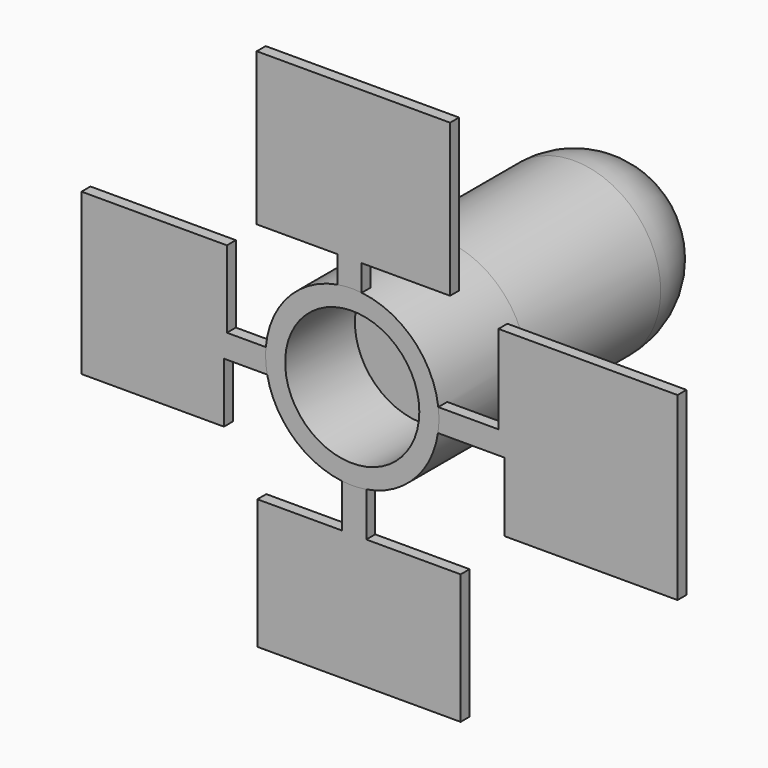
from build123d import *

# Parameters (mm, degrees)
F0_R      = 7.75
F0_R_2    = 5.75
F1_DEPTH  = 7.75
F2_R      = 7.74999
F3_DEPTH  = 15
F4_DEPTH  = 5
F6_R      = 7.75
F6_R_2    = 6
F7_DEPTH  = 9.8
F6_R_3    = 5.75
F8_DEPTH  = 2
F10_DEPTH = 1


# Not quite as in the source:
# - a fillet or chamfer that OpenCascade refuses, or shapes differently, is made with other operations: its cross-section is extruded or revolved along the edge and cut away or added
# - a fillet or chamfer is up to 0.001 mm smaller than in the source, because OpenCascade refuses the exact size


with BuildPart() as f1:
    # F0 (on Front) → F1 (new body)
    with BuildSketch(Plane.XZ):
        Circle(F0_R)
        Circle(F0_R_2, mode=Mode.SUBTRACT)
        Circle(F0_R_2)
    extrude(amount=-F1_DEPTH)

    # F2 (radius 7.75 in the source; OpenCascade refuses exactly that, so slightly less here)
    f2_edges = [f1.edges().sort_by_distance(p)[0] for p in [
        (-7.75, 7.75, 0),
    ]]
    fillet(f2_edges, radius=F2_R)

    # F0 (on Front) → F3 (join)
    with BuildSketch(Plane.XZ):
        Circle(F0_R)
        Circle(F0_R_2, mode=Mode.SUBTRACT)
    extrude(amount=F3_DEPTH)

    # F0 (on Front) → F4 (cut)
    with BuildSketch(Plane.XZ):
        Circle(F0_R_2)
    extrude(amount=-F4_DEPTH, mode=Mode.SUBTRACT)

    # F5: fillet of radius 5.75 on 1 edges, made by hand

    # F5_s1 → F5_t2 (revolve)
    with BuildSketch(Plane.XY):
        with BuildLine():
            ThreePointArc((5.7501, -0.7499), (4.0659639918, 3.3159639918), (0.0001, 5.0001))
            Line((0.0001, 5.0001), (0.0001, 5.1151))
            ThreePointArc((0.0001, 5.1151), (2.87505, 5.115), (5.75, 5.115))
            Line((5.75, 5.115), (5.865, 5))
            ThreePointArc((5.865, 5), (5.865, 2.12505), (5.8651, -0.7499))
            Line((5.8651, -0.7499), (5.7501, -0.7499))
        make_face()
    revolve(axis=Axis((0, 5, 0), (0, -1, 0)))

    # F6 (on face) → F7 (join)
    with BuildSketch(Plane.XZ.offset(15)):
        Circle(F6_R)
        Circle(F6_R_2, mode=Mode.SUBTRACT)
    extrude(amount=F7_DEPTH)

    # F6 (on face) → F8 (join)
    with BuildSketch(Plane.XZ.offset(15)):
        Circle(F6_R_2)
        Circle(F6_R_3, mode=Mode.SUBTRACT)
        Circle(F6_R_3)
    extrude(amount=F8_DEPTH)

    # F9 (on face) → F10 (join)
    with BuildSketch(Plane.XZ.offset(24.8)):
        with BuildLine():
            ThreePointArc((-7.6053065566, -1.4905744465), (-7.7379420075, -0.4321498454), (-7.7239859171, 0.6344616239))
            Line((-7.7239859171, 0.6344616239), (-11.2089226057, 0.6344616239))
            Line((-11.2089226057, 0.6344616239), (-11.2089226057, 7.51422951))
            Line((-11.2089226057, 7.51422951), (-24.211389944, 7.51422951))
            Line((-24.211389944, 7.51422951), (-24.211389944, -6.8491166458))
            Line((-24.211389944, -6.8491166458), (-11.4740878344, -6.8491166458))
            Line((-11.4740878344, -6.8491166458), (-11.4740878344, -1.4905744465))
            Line((-11.4740878344, -1.4905744465), (-7.6053065566, -1.4905744465))
        make_face()
        with BuildLine():
            ThreePointArc((-1.3181141258, 7.6370855142), (-0.2358353441, 7.7464108909), (0.8510895829, 7.7031257631))
            Line((0.8510895829, 7.7031257631), (0.8510895829, 10.0341412146))
            Line((0.8510895829, 10.0341412146), (8.7516037747, 10.0341412146))
            Line((8.7516037747, 10.0341412146), (8.7516037747, 23.6629825085))
            Line((8.7516037747, 23.6629825085), (-8.5408838931, 23.6629825085))
            Line((-8.5408838931, 23.6629825085), (-8.5408838931, 10.2677652612))
            Line((-8.5408838931, 10.2677652612), (-8.5408838931, 10.0341412146))
            Line((-8.5408838931, 10.0341412146), (-1.3181141258, 10.0341412146))
            Line((-1.3181141258, 10.0341412146), (-1.3181141258, 7.6370855142))
        make_face()
        with BuildLine():
            Line((13.07656436, 0.9255647358), (7.6945324692, 0.9255647358))
            ThreePointArc((7.6945324692, 0.9255647358), (7.7361206892, 0.463612642), (7.75, 0))
            ThreePointArc((7.75, 0), (7.7293938157, -0.5647753903), (7.6676848409, -1.1265474604))
            Line((7.6676848409, -1.1265474604), (13.6271854863, -1.1265474604))
            Line((13.6271854863, -1.1265474604), (13.6271854863, -7.3085245676))
            Line((13.6271854863, -7.3085245676), (29.0946420282, -7.3085245676))
            Line((29.0946420282, -7.3085245676), (29.0946420282, 8.8346945122))
            Line((29.0946420282, 8.8346945122), (13.07656436, 8.8346945122))
            Line((13.07656436, 8.8346945122), (13.07656436, 0.9255647358))
        make_face()
        with BuildLine():
            Line((1.256284304, -11.5922550619), (1.256284304, -7.6474995749))
            ThreePointArc((1.256284304, -7.6474995749), (0.1659608629, -7.748222828), (-0.9276754413, -7.6942782817))
            Line((-0.9276754413, -7.6942782817), (-0.9276754413, -11.5922550619))
            Line((-0.9276754413, -11.5922550619), (-8.4876073524, -11.5922550619))
            Line((-8.4876073524, -11.5922550619), (-8.4876073524, -23.2104603201))
            Line((-8.4876073524, -23.2104603201), (9.6937846392, -23.2104603201))
            Line((9.6937846392, -23.2104603201), (9.6937846392, -11.5922550619))
            Line((9.6937846392, -11.5922550619), (1.256284304, -11.5922550619))
        make_face()
    extrude(amount=-F10_DEPTH)


solid = f1.part
